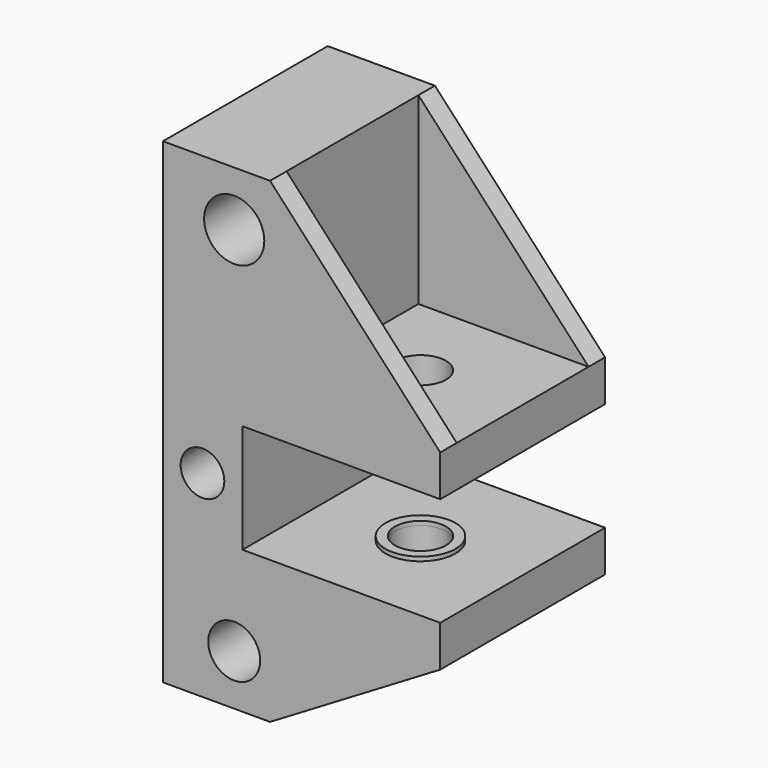
from build123d import *

# Parameters (mm, degrees)
F0_R          = 3.15
F0_R_2        = 3.65
F1_DEPTH      = 25
F2_R          = 3.1
F3_DEPTH      = 17.301
F3_DEPTH_BACK = 40.501
F2_R_2        = 4.25
F4_DEPTH      = 0.5
F5_R          = 4.25
F5_R_2        = 3.1
F6_DEPTH      = 0.5
F7_W          = 20.65
F7_H          = 20
F8_DEPTH      = 22.3
F9_W          = 20.65
F9_H          = 20
F10_DEPTH     = 12.3
F11_R         = 2.65
F12_DEPTH     = 25.001
F13_T         = 2.5
F13_T3_DEPTH  = 27.3
F13_T5_DEPTH  = 25.65
F13_T7_DEPTH  = 30
F13_T9_DEPTH  = 25
F13_T11_DEPTH = 17.3


# Not quite as in the source:
# - a shell that OpenCascade refuses in one call is made with other operations: the cavity is built on its own and cut out


with BuildPart() as f1:
    # F0 (on Front) → F1 (new body)
    with BuildSketch(Plane.XZ):
        Polygon((4.35, 29.15), (-8.65, 29.15), (-8.65, -28.65), (4.35, -28.65), (25, -16.35), (25, -11.35), (1, -11.35), (1, 1.85), (25, 1.85), (25, 6.85), align=None)
        with Locations((0, -22.5)):
            Circle(F0_R, mode=Mode.SUBTRACT)
        with Locations((0, 22.5)):
            Circle(F0_R_2, mode=Mode.SUBTRACT)
    extrude(amount=F1_DEPTH)

    # F2 (on face) → F3 (cut, two sides)
    with BuildSketch(Plane.XY.offset(-11.35)) as f3_sk:
        with Locations((13, -13)):
            Circle(F2_R)
    extrude(amount=-F3_DEPTH, mode=Mode.SUBTRACT)
    extrude(f3_sk.sketch, amount=F3_DEPTH_BACK, mode=Mode.SUBTRACT)

    # F2 (on face) → F4 (join)
    with BuildSketch(Plane.XY.offset(-11.35)):
        with Locations((13, -13)):
            Circle(F2_R_2)
        with Locations((13, -13)):
            Circle(F2_R, mode=Mode.SUBTRACT)
    extrude(amount=F4_DEPTH)

    # F5 (on face) → F6 (join)
    with BuildSketch(Plane(origin=(0, 0, 1.85), x_dir=(1, 0, 0), z_dir=(0, 0, -1))):
        with Locations((13, 13)):
            Circle(F5_R)
        with Locations((13, 13)):
            Circle(F5_R_2, mode=Mode.SUBTRACT)
    extrude(amount=F6_DEPTH)

    # F7 (on face) → F8 (cut)
    with BuildSketch(Plane.XY.offset(29.15)):
        with Locations((14.675, -12.5)):
            Rectangle(F7_W, F7_H)
    extrude(amount=-F8_DEPTH, mode=Mode.SUBTRACT)

    # F9 (on face) → F10 (cut)
    with BuildSketch(Plane(origin=(0, 0, -28.65), x_dir=(1, 0, 0), z_dir=(0, 0, -1))):
        with Locations((14.675, 12.5)):
            Rectangle(F9_W, F9_H)
    extrude(amount=-F10_DEPTH, mode=Mode.SUBTRACT)

    # F11 (on face) → F12 (cut, through all)
    with BuildSketch(Plane.XZ.offset(25)):
        with Locations((-3.85, -4.75)):
            Circle(F11_R)
    extrude(amount=-F12_DEPTH, mode=Mode.SUBTRACT)

    # F13: shell of thickness 2.5, made by hand


with BuildPart() as f13_core1:
    # F13_t2: copy of F1
    add(f1.part)

    # the walls: a layer under each face that stays
    f13_faces = [f13_core1.faces().sort_by_distance(p)[0] for p in [
        (14.675, -1.25, 18),
        (-3.0416666667, 0, -19.0166666667),
        (-2.15, -12.5, 29.15),
        (14.675, -2.5, 10.5666666667),
        (25, -12.5, 4.35),
        (5, -20.8333333333, 1.85),
        (1, -12.5, -4.75),
        (-2.15, -12.5, -28.65),
        (21, -20.8333333333, -11.35),
        (14.675, -1.25, -22.5),
        (25, -12.5, -13.85),
        (-6.5, -12.5, -4.75),
        (-3.15, -12.5, -22.5),
        (-3.65, -12.5, 22.5),
        (4.35, -12.5, 18),
        (14.675, -23.75, 18),
        (-3.0416666667, -25, -19.0166666667),
        (7.7916666667, -19.1666666667, 6.85),
        (8.75, -13, 1.6),
        (4.35, -12.5, -22.5),
        (14.675, -23.75, -22.5),
        (8.75, -13, -11.1),
        (7.7916666667, -2.5, -18.4),
        (7.7916666667, -5.8333333333, -16.35),
        (7.7916666667, -22.5, 10.5666666667),
        (9.9, -13, 4.35),
        (10.1666666667, -10.1666666667, 1.35),
        (14.675, -22.5, -18.4),
        (10.1666666667, -15.8333333333, -10.85),
        (9.9, -13, -13.85),
        (9.9, -13, 1.6),
        (9.9, -13, -11.1),
    ]]
    thicken(f13_faces, amount=-F13_T, mode=Mode.SUBTRACT)

    # F13_s4 → F13_t3 (cut)
    with BuildSketch(Plane.XY.offset(4.35)):
        Polygon((4.375, -2.525), (4.35, 0), (1.85, 0), (1.85, -2.5), align=None)
        Polygon((4.375, -22.475), (1.85, -22.5), (1.85, -25), (4.35, -25), align=None)
    extrude(amount=F13_T3_DEPTH, mode=Mode.SUBTRACT)

    # F13_s6 → F13_t5 (cut)
    with BuildSketch(Plane.YZ.offset(1.85)):
        Polygon((-2.525, 6.875), (0, 6.85), (0, 4.35), (-2.5, 4.35), align=None)
        Polygon((-22.475, 6.875), (-22.5, 4.35), (-25, 4.35), (-25, 6.85), align=None)
        Polygon((-2.525, -16.375), (0, -16.35), (0, -13.85), (-2.5, -13.85), align=None)
        Polygon((-22.475, -16.375), (-22.5, -13.85), (-25, -13.85), (-25, -16.35), align=None)
    extrude(amount=F13_T5_DEPTH, mode=Mode.SUBTRACT)

    # F13_s8 → F13_t7 (cut)
    with BuildSketch(Plane.XZ.offset(-2.5)):
        Polygon((1.025, 1.825), (1, 4.35), (-1.5, 4.35), (-1.5, 1.85), align=None)
        Polygon((1.025, -11.325), (-1.5, -11.35), (-1.5, -13.85), (1, -13.85), align=None)
    extrude(amount=F13_T7_DEPTH, mode=Mode.SUBTRACT)

    # F13_s10 → F13_t9 (cut)
    with BuildSketch(Plane.XZ):
        Polygon((4.375, 6.875), (1.85, 6.85), (1.85, 4.35), (4.35, 4.35), align=None)
        Polygon((4.375, -16.375), (1.85, -16.35), (1.85, -13.85), (4.35, -13.85), align=None)
    extrude(amount=F13_T9_DEPTH, mode=Mode.SUBTRACT)

    # F13_s12 → F13_t11 (cut)
    with BuildSketch(Plane.XY.offset(-31.15)):
        Polygon((4.375, -22.475), (1.85, -22.5), (1.85, -25), (4.35, -25), align=None)
        Polygon((4.375, -2.525), (1.85, -2.5), (1.85, 0), (4.35, 0), align=None)
    extrude(amount=F13_T11_DEPTH, mode=Mode.SUBTRACT)

    # F13_s13 → F13_t14 (revolve, cut)
    with BuildSketch(Plane.XZ.offset(13)):
        Polygon((17.275, 1.825), (17.25, 4.35), (14.75, 4.35), (14.75, 1.85), align=None)
    revolve(axis=Axis((13, -13, 1.85), (0, 0, -1)), mode=Mode.SUBTRACT)

    # F13_s15 → F13_t16 (revolve, cut)
    with BuildSketch(Plane.XZ.offset(13)):
        Polygon((17.275, -11.325), (17.25, -13.85), (14.75, -13.85), (14.75, -11.35), align=None)
    revolve(axis=Axis((13, -13, -11.35), (0, 0, 1)), mode=Mode.SUBTRACT)


with BuildPart() as f1_1:
    add(f1.part)

    # what is left inside the walls is the cavity
    f13_cavity = [f13_core1.part.solids().sort_by_distance(p)[0] for p in [
        (-8.625, -15.833333, 11.883073),
        (-8.625, -15.833333, -16.383073),
    ]]
    add(f13_cavity, mode=Mode.SUBTRACT)


solid = f1_1.part
